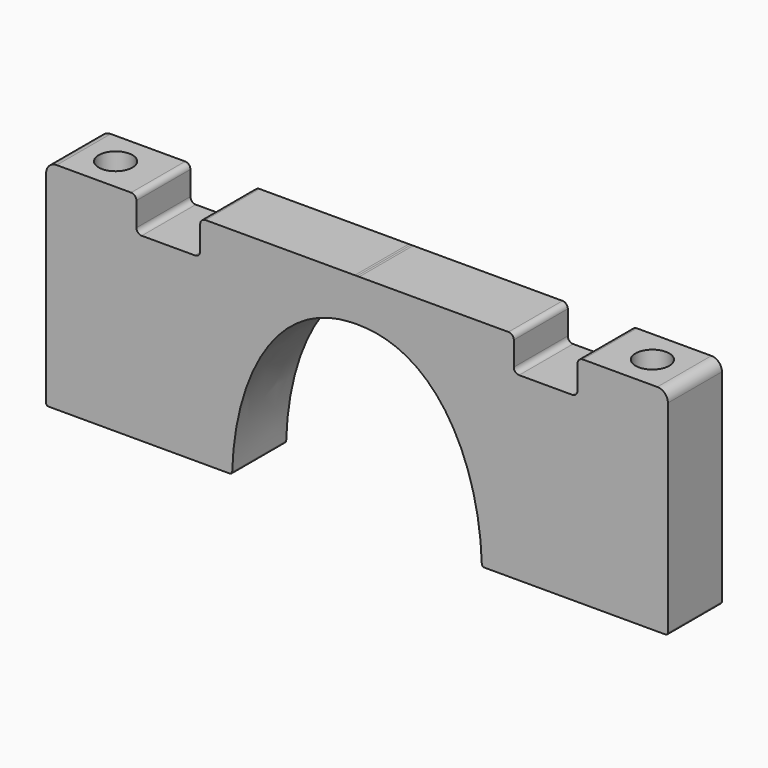
from build123d import *

# Parameters (mm, degrees)
F1_DEPTH = 12.7
F2_R     = 3.175
F3_DEPTH = 41.5002601562
F4_W     = 130.419023335
F4_H     = 4.1049833633
F5_DEPTH = 25
F6_R     = 2
F7_R     = 0.432
F9_DEPTH = 12.7
F10_R    = 1


# Not quite as in the source:
# - ends of sketch curves that miss each other by under 0.0002 mm in the source are joined
# - the dataset's text gives a spline's control points without its knots; the knots are read off the source's solid


with BuildPart() as f1:
    # F0 (on Front) → F1 (new body)
    with BuildSketch(Plane.XZ):
        with BuildLine():
            Line((-8, 0), (0, 0))
            add(Edge.make_bspline(
                [(0, 0), (0, 16.0348825157), (7.430841215, 33.6514413357), (23.5, 33.5)],
                knots=[0, 0, 0, 0, 40.9206549312, 40.9206549312, 40.9206549312, 40.9206549312], degree=3))
            add(Edge.make_bspline(
                [(47, 0), (47, 16.0348825157), (39.569158785, 33.6514413357), (23.5, 33.5)],
                knots=[0, 0, 0, 0, 40.9206549312, 40.9206549312, 40.9206549312, 40.9206549312], degree=3))
            Line((47, 0), (55, 0))
            add(Edge.make_bspline(
                [(55, 0), (55, 2.3133051501), (54.8084752548, 5.6604865088), (54.3346414744, 8.9941225704), (54.1644875118, 10.0000161913)],
                knots=[0, 0, 0, 0, 0.125, 0.1792883855, 0.1792883855, 0.1792883855, 0.1792883855], degree=3))
            add(Edge.make_bspline(
                [(54.1644875118, 10.0000161913), (53.9428588652, 11.3102110198), (53.2041802455, 14.9199242801), (51.403557473, 20.6965522199), (48.312647429, 27.0635606249), (44.7757382973, 31.8590791464), (41.27501086, 35.2044913237), (38.3020149436, 37.39930019), (34.9881581098, 39.2038242784), (31.3670929719, 40.5407901401), (27.6491274865, 41.3170292606), (25.11417344, 41.4919330376), (23.9092731988, 41.5002601562)],
                knots=[0.1792883855, 0.1792883855, 0.1792883855, 0.1792883855, 0.25, 0.375, 0.5, 0.625, 0.6875, 0.75, 0.8125, 0.875, 0.9375, 0.9926226885, 0.9926226885, 0.9926226885, 0.9926226885], degree=3))
            Line((23.9092731988, 41.5002601562), (23.5, 41.5002601562))
            Line((23.5, 41.5002601562), (23.0907268012, 41.5002601562))
            add(Edge.make_bspline(
                [(-7.1644875118, 10.0000161913), (-6.9428588652, 11.3102110198), (-6.2041802455, 14.9199242801), (-4.403557473, 20.6965522199), (-1.312647429, 27.0635606249), (2.2242617027, 31.8590791464), (5.72498914, 35.2044913237), (8.6979850564, 37.39930019), (12.0118418902, 39.2038242784), (15.6329070281, 40.5407901401), (19.3508725135, 41.3170292606), (21.88582656, 41.4919330376), (23.0907268012, 41.5002601562)],
                knots=[0.1792883855, 0.1792883855, 0.1792883855, 0.1792883855, 0.25, 0.375, 0.5, 0.625, 0.6875, 0.75, 0.8125, 0.875, 0.9375, 0.9926226885, 0.9926226885, 0.9926226885, 0.9926226885], degree=3))
            add(Edge.make_bspline(
                [(-8, 0), (-8, 2.3133051501), (-7.8084752548, 5.6604865088), (-7.3346414744, 8.9941225704), (-7.1644875118, 10.0000161913)],
                knots=[0, 0, 0, 0, 0.125, 0.1792883855, 0.1792883855, 0.1792883855, 0.1792883855], degree=3))
        make_face()
        with BuildLine():
            Line((-35, 0), (-8, 0))
            add(Edge.make_bspline(
                [(-8, 0), (-8, 2.3133051501), (-7.8084752548, 5.6604865088), (-7.3346414744, 8.9941225704), (-7.1644875118, 10.0000161913)],
                knots=[0, 0, 0, 0, 0.125, 0.1792883855, 0.1792883855, 0.1792883855, 0.1792883855], degree=3))
            Line((-7.1644875118, 10.0000161913), (-35, 10))
            Line((-35, 10), (-35, 0))
        make_face()
        with BuildLine():
            Line((-35, 10), (-7.1643917939, 10))
            add(Edge.make_bspline(
                [(-7.1643917939, 10), (-6.9428588652, 11.3102110198), (-6.2041802455, 14.9199242801), (-4.403557473, 20.6965522199), (-1.312647429, 27.0635606249), (2.2242617027, 31.8590791464), (5.72498914, 35.2044913237), (8.6979850564, 37.39930019), (12.0118418902, 39.2038242784), (15.6329070281, 40.5407901401), (19.3508725135, 41.3170292606), (21.88582656, 41.4919330376), (23.0907268012, 41.5002601562)],
                knots=[0.1792883855, 0.1792883855, 0.1792883855, 0.1792883855, 0.25, 0.375, 0.5, 0.625, 0.6875, 0.75, 0.8125, 0.875, 0.9375, 0.9926226885, 0.9926226885, 0.9926226885, 0.9926226885], degree=3))
            Line((23.0907268012, 41.5002601562), (-12, 41.5002601562))
            Line((-12, 41.5002601562), (-12, 38.0002601562))
            Line((-12, 38.0002601562), (-15, 38.0002601562))
            Line((-15, 38.0002601562), (-18, 38.0002601562))
            Line((-18, 38.0002601562), (-18, 41.5002601562))
            Line((-18, 41.5002601562), (-35, 41.5002601562))
            Line((-35, 41.5002601562), (-35, 10))
        make_face()
        with BuildLine():
            add(Edge.make_bspline(
                [(55, 0), (55, 2.3133051501), (54.8084752548, 5.6604865088), (54.3346414744, 8.9941225704), (54.1644875118, 10.0000161913)],
                knots=[0, 0, 0, 0, 0.125, 0.1792883855, 0.1792883855, 0.1792883855, 0.1792883855], degree=3))
            Line((55, 0), (82, 0))
            Line((82, 0), (82, 10))
            Line((82, 10), (54.1644875118, 10.0000161913))
        make_face()
        with BuildLine():
            add(Edge.make_bspline(
                [(23.0907268012, 41.5002601562), (23.2269381476, 41.5012015188), (23.3633657228, 41.5012017791), (23.499999998, 41.5002598872)],
                knots=[0.9926226885, 0.9926226885, 0.9926226885, 0.9926226885, 0.9988541884, 0.9988541884, 0.9988541884, 0.9988541884], degree=3))
            Line((23.0907268012, 41.5002601562), (23.499999998, 41.5002598872))
        make_face()
        with BuildLine():
            add(Edge.make_bspline(
                [(54.1644875118, 10.0000161913), (53.9428588652, 11.3102110198), (53.2041802455, 14.9199242801), (51.403557473, 20.6965522199), (48.312647429, 27.0635606249), (44.7757382973, 31.8590791464), (41.27501086, 35.2044913237), (38.3020149436, 37.39930019), (34.9881581098, 39.2038242784), (31.3670929719, 40.5407901401), (27.6491274865, 41.3170292606), (25.11417344, 41.4919330376), (23.9092731988, 41.5002601562)],
                knots=[0.1792883855, 0.1792883855, 0.1792883855, 0.1792883855, 0.25, 0.375, 0.5, 0.625, 0.6875, 0.75, 0.8125, 0.875, 0.9375, 0.9926226885, 0.9926226885, 0.9926226885, 0.9926226885], degree=3))
            Line((54.1644875118, 10.0000161913), (82, 10))
            Line((82, 10), (82, 41.5002601562))
            Line((82, 41.5002601562), (23.9092731988, 41.5002601562))
        make_face()
        with BuildLine():
            add(Edge.make_bspline(
                [(23.9092731988, 41.5002601562), (23.7730618524, 41.5012015188), (23.6366342772, 41.5012017791), (23.500000002, 41.5002598872)],
                knots=[0.9926226885, 0.9926226885, 0.9926226885, 0.9926226885, 0.9988541884, 0.9988541884, 0.9988541884, 0.9988541884], degree=3))
            Line((23.500000002, 41.5002598872), (23.9092731988, 41.5002601562))
        make_face()
        Polygon((-12, 38.0002601562), (-12, 41.5002601562), (-15, 41.5002601562), (-18, 41.5002601562), (-18, 38.0002601562), (-15, 38.0002601562), align=None)
    extrude(amount=F1_DEPTH)

    # F2 (on face) → F3 (cut, through all)
    with BuildSketch(Plane.XY.offset(41.5002601562)):
        with Locations((-26.999999998, -6.35)):
            Circle(F2_R)
        with Locations((74.000000002, -6.35)):
            Circle(F2_R)
    extrude(amount=-F3_DEPTH, mode=Mode.SUBTRACT)

    # F4 (on Front) → F5 (cut)
    with BuildSketch(Plane.XZ):
        with Locations((22.7671675384, -1.0524916817)):
            Rectangle(F4_W, F4_H)
    extrude(amount=F5_DEPTH, mode=Mode.SUBTRACT)

    # F6
    f6_edges = [f1.edges().sort_by_distance(p)[0] for p in [
        (82, -6.35, 41.50026),
        (-35, -6.35, 41.50026),
    ]]
    fillet(f6_edges, radius=F6_R)

    # F7
    f7_edges = [f1.edges().sort_by_distance(p)[0] for p in [
        (-35, -6.35, 1),
        (0.009608, -6.35, 1),
        (46.990392, -6.35, 1),
        (82, -6.35, 1),
    ]]
    fillet(f7_edges, radius=F7_R)

    # F8 (on face) → F9 (cut, through all)
    with BuildSketch(Plane.XZ.offset(12.7)):
        Polygon((-18, 35.0002601562), (-12, 35.0002601562), (-6, 35.0002601562), (-6, 41.5002601562), (-12, 41.5002601562), (-18, 41.5002601562), align=None)
        Polygon((59.0000000039, 35.0002601562), (65.0000000039, 35.0002601562), (65.0000000039, 41.5002601562), (59.0000000039, 41.5002601562), (53.0000000039, 41.5002601562), (53.0000000039, 35.0002601562), align=None)
    extrude(amount=-F9_DEPTH, mode=Mode.SUBTRACT)

    # F10
    f10_edges = [f1.edges().sort_by_distance(p)[0] for p in [
        (-18, -6.35, 35.00026),
        (-6, -6.35, 35.00026),
        (-18, -6.35, 41.50026),
        (-6, -6.35, 41.50026),
        (53, -6.35, 35.00026),
        (53, -6.35, 41.50026),
        (65, -6.35, 35.00026),
        (65, -6.35, 41.50026),
    ]]
    fillet(f10_edges, radius=F10_R)


solid = f1.part
